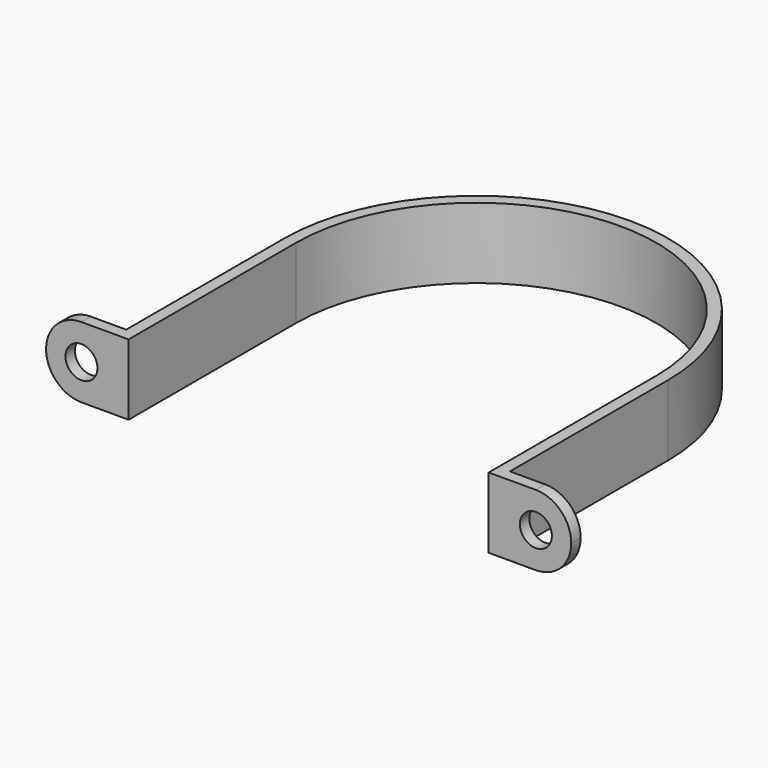
from build123d import *

# Parameters (mm, degrees)
F1_DEPTH = 9.525
F2_R     = 4.76249
F3_R     = 2.15265
F4_DEPTH = 1.5875


# Not quite as in the source:
# - a fillet or chamfer is up to 0.001 mm smaller than in the source, because OpenCascade refuses the exact size


with BuildPart() as f1:
    # F0 (on Top) → F1 (new body)
    with BuildSketch(Plane.XY):
        with BuildLine():
            Line((-24.257, -28.2194), (-24.257, 0))
            ThreePointArc((-24.257, 0), (0, 24.257), (24.257, 0))
            Line((24.257, 0), (24.257, -28.2194))
            Line((24.257, -28.2194), (35.3695, -28.2194))
            Line((35.3695, -28.2194), (35.3695, -26.6319))
            Line((35.3695, -26.6319), (25.8445, -26.6319))
            Line((25.8445, -26.6319), (25.8445, 0))
            ThreePointArc((25.8445, 0), (0, 25.8445), (-25.8445, 0))
            Line((-25.8445, 0), (-25.8445, -26.6319))
            Line((-25.8445, -26.6319), (-35.3695, -26.6319))
            Line((-35.3695, -26.6319), (-35.3695, -28.2194))
            Line((-35.3695, -28.2194), (-24.257, -28.2194))
        make_face()
    extrude(amount=F1_DEPTH)

    # F2 (radius 4.7625 in the source; OpenCascade refuses exactly that, so slightly less here)
    f2_edges = [f1.edges().sort_by_distance(p)[0] for p in [
        (35.3695, -27.42565, 9.525),
        (35.3695, -27.42565, 0),
        (-35.3695, -27.42565, 0),
        (-35.3695, -27.42565, 9.525),
    ]]
    fillet(f2_edges, radius=F2_R)

    # F3 (on face) → F4 (cut, through all)
    with BuildSketch(Plane.XZ.offset(28.2194)):
        with Locations((30.607, 4.7625)):
            Circle(F3_R)
        with Locations((-30.607, 4.7625)):
            Circle(F3_R)
    extrude(amount=-F4_DEPTH, mode=Mode.SUBTRACT)


solid = f1.part
